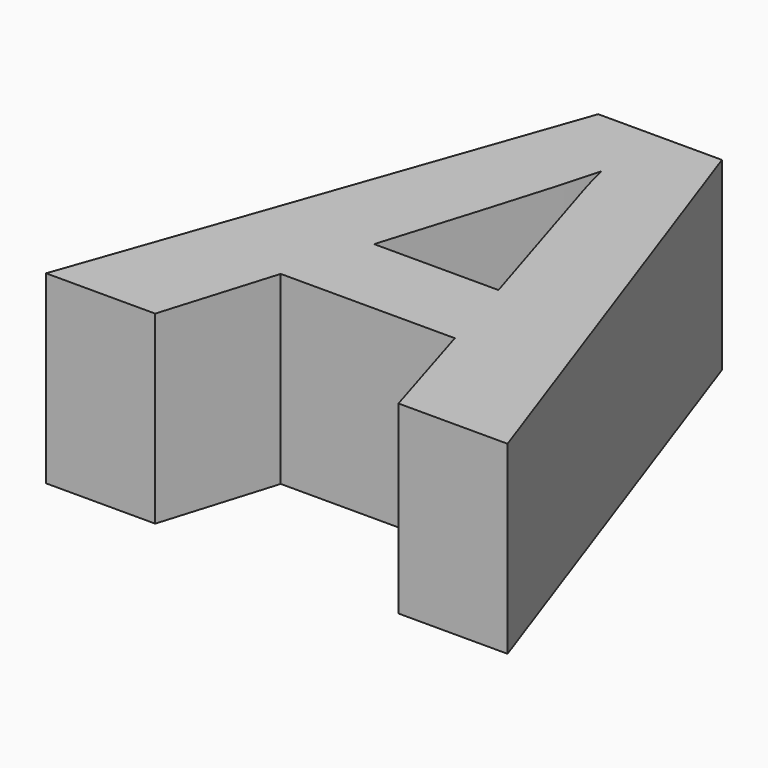
from build123d import *

# Parameters (mm, degrees)
F0_TEXT_SIZE = 91.8633304536
F1_DEPTH     = 25.4


# Not quite as in the source:
# - Text() gives the source's letters only with a copy of the font that has no kerning and outlines rounded to 1/6400 em; it was checked with that copy


with BuildPart() as f1:
    # F0 (on Top) → F1 (new body)
    with BuildSketch(Plane.XY):
        with Locations((-31.915102154, -28.3591002226)):
            Text('A', F0_TEXT_SIZE, font='Open Sans', font_style=FontStyle.BOLD, text_align=(TextAlign.LEFT, TextAlign.BOTTOM))
    extrude(amount=F1_DEPTH)


solid = f1.part
